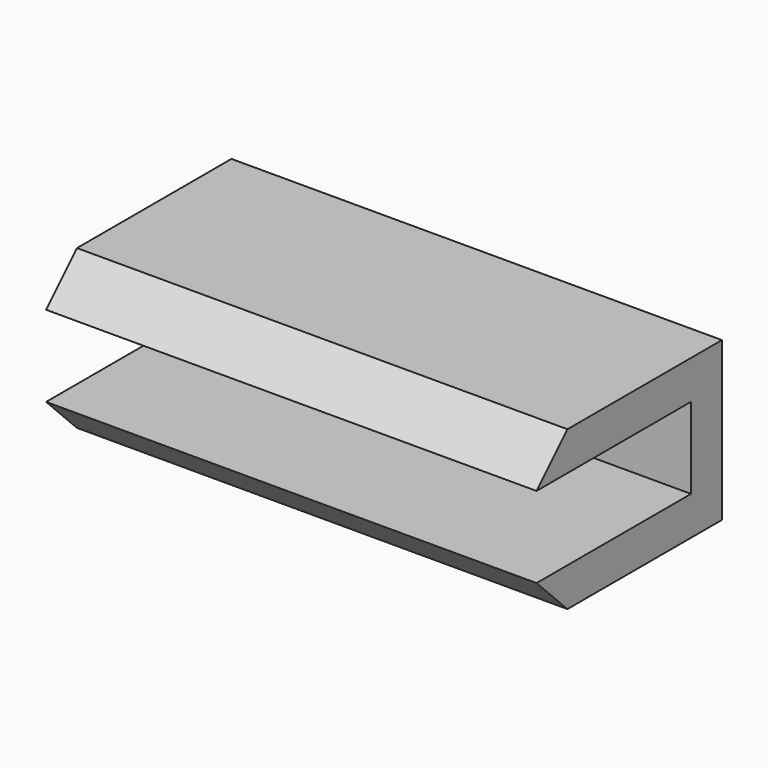
from build123d import *

# Parameters (mm, degrees)
F0_W     = 63.5
F0_H     = 5
F1_DEPTH = 10.5
F2_W     = 63.5
F2_H     = 25
F2_H_2   = 5
F3_DEPTH = 5
F4_SIZE  = 4.99999
F5_W     = 63.5
F5_H     = 5
F5_H_2   = 25
F6_DEPTH = 5
F7_SIZE  = 4.99999


# Not quite as in the source:
# - a fillet or chamfer is up to 0.001 mm smaller than in the source, because OpenCascade refuses the exact size


with BuildPart() as f1:
    # F0 (on Top) → F1 (new body)
    with BuildSketch(Plane.XY):
        Rectangle(F0_W, F0_H)
    extrude(amount=F1_DEPTH)

    # F2 (on face) → F3 (join)
    with BuildSketch(Plane.XY.offset(10.5)):
        with Locations((0, -15)):
            Rectangle(F2_W, F2_H)
        Rectangle(F2_W, F2_H_2)
    extrude(amount=F3_DEPTH)

    # F4 (size 5 in the source; OpenCascade refuses exactly that, so slightly less here)
    f4_edges = [f1.edges().sort_by_distance(p)[0] for p in [
        (0, -27.5, 15.5),
    ]]
    chamfer(f4_edges, length=F4_SIZE)

    # F5 (on face) → F6 (join)
    with BuildSketch(Plane(origin=(0, 0, 0), x_dir=(1, 0, 0), z_dir=(0, 0, -1))):
        Rectangle(F5_W, F5_H)
        with Locations((0, 15)):
            Rectangle(F5_W, F5_H_2)
    extrude(amount=F6_DEPTH)

    # F7 (size 5 in the source; OpenCascade refuses exactly that, so slightly less here)
    f7_edges = [f1.edges().sort_by_distance(p)[0] for p in [
        (0, -27.5, -5),
    ]]
    chamfer(f7_edges, length=F7_SIZE)


solid = f1.part
